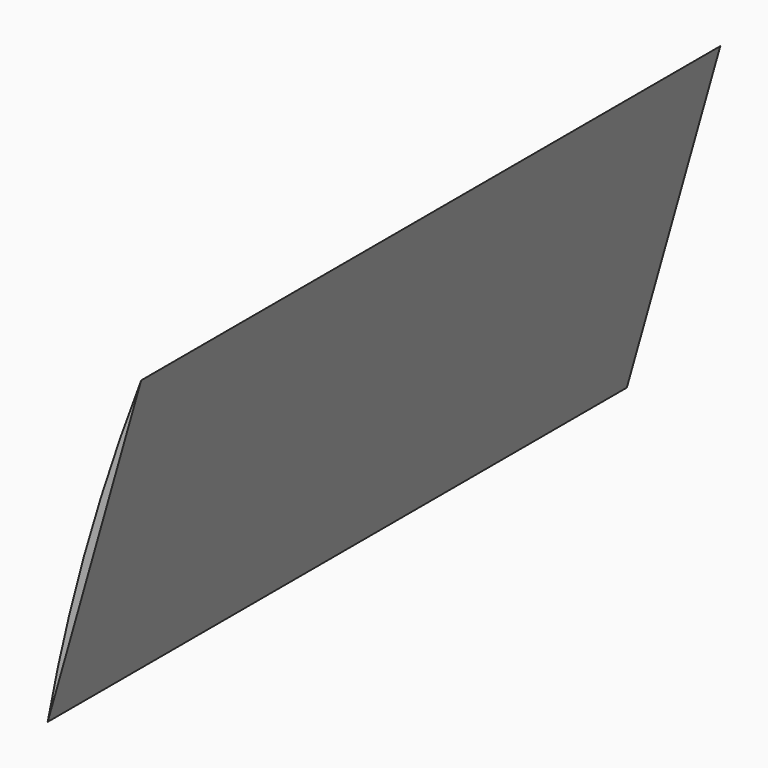
from build123d import *

# Parameters (mm, degrees)
F4_DEPTH = 25


with BuildPart() as f4:
    # F3 (on Front) → F4 (new body)
    with BuildSketch(Plane.XZ):
        with BuildLine():
            add(Edge.make_bspline(
                [(3.2284122208, -209.6570315379), (2.1661361953, -213.437092478), (1.0892706333, -217.2493781635), (0, -221.0912411008)],
                knots=[0.9755503587, 0.9755503587, 0.9755503587, 0.9755503587, 1, 1, 1, 1], degree=3))
            add(Edge.make_bspline(
                [(3.2284122208, -209.6570315379), (1.7847289061, -213.4491712031), (0.695584279, -217.2596157222), (0, -221.0912411008)],
                knots=[378.6006558751, 378.6006558751, 378.6006558751, 378.6006558751, 390.9679300919, 390.9679300919, 390.9679300919, 390.9679300919], degree=3))
        make_face()
    extrude(amount=F4_DEPTH)


solid = f4.part
